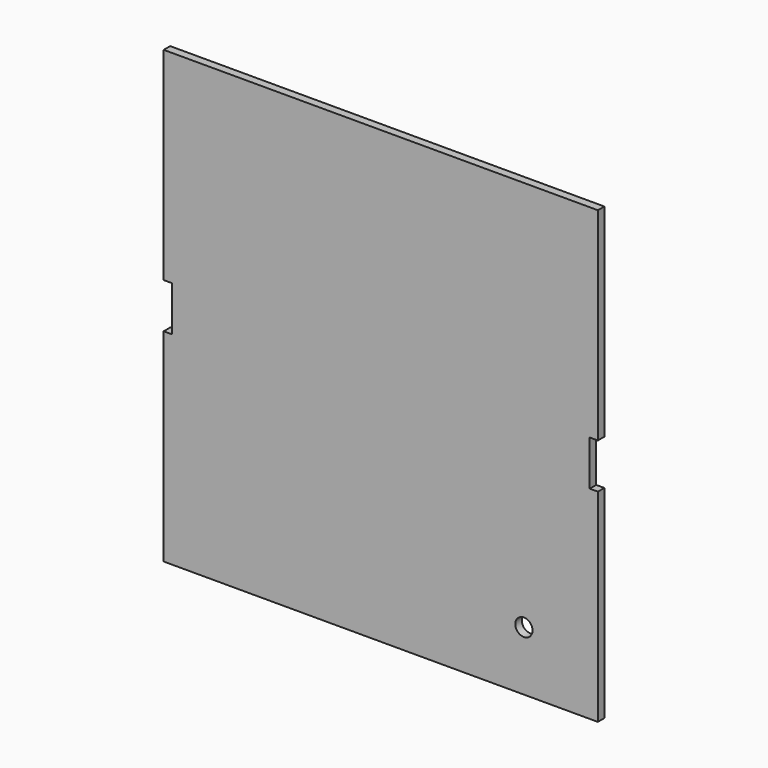
from build123d import *

# Parameters (mm, degrees)
F0_R     = 2.921
F1_DEPTH = 2.7432


# Not quite as in the source:
# - a feature names something its author has since deleted; it is built from what else it names


with BuildPart() as f1:
    # F0 (on Front) → F1 (new body)
    with BuildSketch(Plane.XZ):
        Polygon((-15.24, 118.095377792), (-81.0768, 118.095377792), (-81.0768, 49.515377792), (-78.3336, 49.515377792), (-78.3336, 34.275377792), (-81.0768, 34.275377792), (-81.0768, -34.304622208), (-15.24, -34.304622208), (0, -34.304622208), (65.8114, -34.304622208), (65.8114, 34.275377792), (63.0682, 34.275377792), (63.0682, 49.515377792), (65.8114, 49.515377792), (65.8114, 118.095377792), (0, 118.095377792), align=None)
        with Locations((40.7993271947, -14.2451748252)):
            Circle(F0_R, mode=Mode.SUBTRACT)
    extrude(amount=F1_DEPTH)


solid = f1.part
